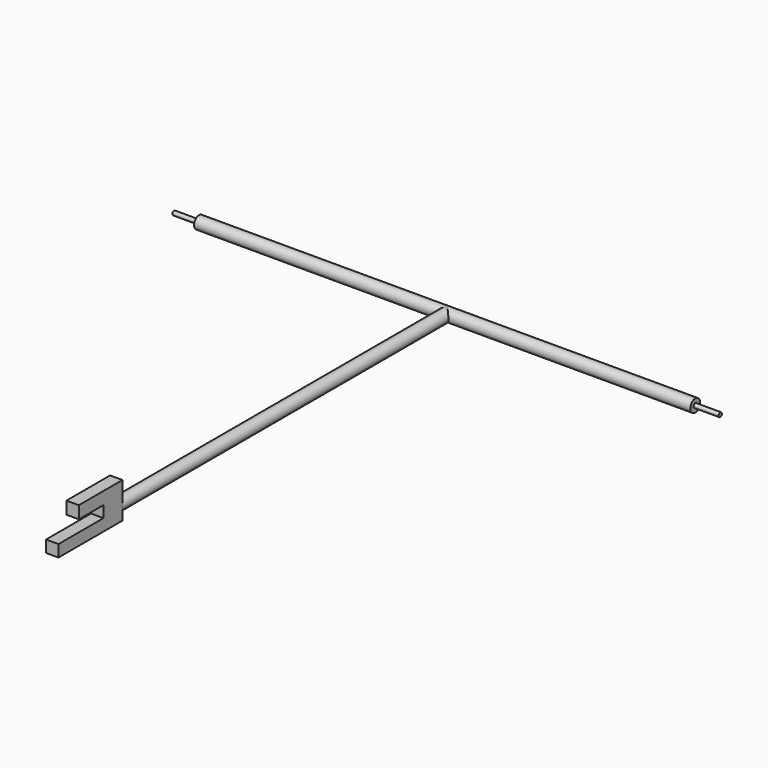
from build123d import *

# Parameters (mm, degrees)
F2_R      = 0.75
F10_R     = 0.25
F15_R     = 0.75
F19_DEPTH = 0.75


# Not quite as in the source:
# - a feature of the source that left no trace in its solid (it failed there, or was rolled back) is left out
# - a pattern or mirror of a feature is missing from the dataset's text; its kind, count and spacing are read off the source's solid


with BuildPart() as f3:
    # F3: sweep along a path in F0
    with BuildLine(Plane.XZ) as f3_path:
        Line((-30, 0), (0, 0))
        Line((0, 0), (30, 0))
    # F2 (on plane+point) → F3 (sweep)
    with BuildSketch(Plane.YZ.offset(-30)):
        Circle(F2_R)
    sweep(path=f3_path.line)

    # F11: sweep along a path in F8
    with BuildLine(Plane.XZ) as f11_path:
        Line((0, 0), (33.02, 0))
    # F10 (on plane+point) → F11 (sweep)
    with BuildSketch(Plane.YZ.offset(33.02)):
        Circle(F10_R)
    f11 = sweep(path=f11_path.line)

    # F11_copies: F11 across plane
    add(f11.mirror(Plane(origin=(-0.001764, 0, 0), x_dir=(0, 0, -1), z_dir=(-1, 0, 0))))

    # F16: sweep along a path in F13
    with BuildLine(Plane.YZ) as f16_path:
        Line((0, 0), (-50, 0))
    # F15 (on plane+point) → F16 (sweep)
    with BuildSketch(Plane.XZ.offset(50)):
        Circle(F15_R)
    sweep(path=f16_path.line)

    # F18 (on plane+point) → F19 (join, symmetric)
    with BuildSketch(Plane.YZ):
        Polygon((-50, -1.4374784192), (-50, 0), (-50, 2.8882389888), (-56.6018782556, 2.8882389888), (-56.6018782556, 1.3868947281), (-52.8817437589, 1.3868947281), (-52.8817437589, 0), (-59.6723221242, 0), (-59.6723221242, -1.4374784192), align=None)
    extrude(amount=F19_DEPTH, both=True)


solid = f3.part
